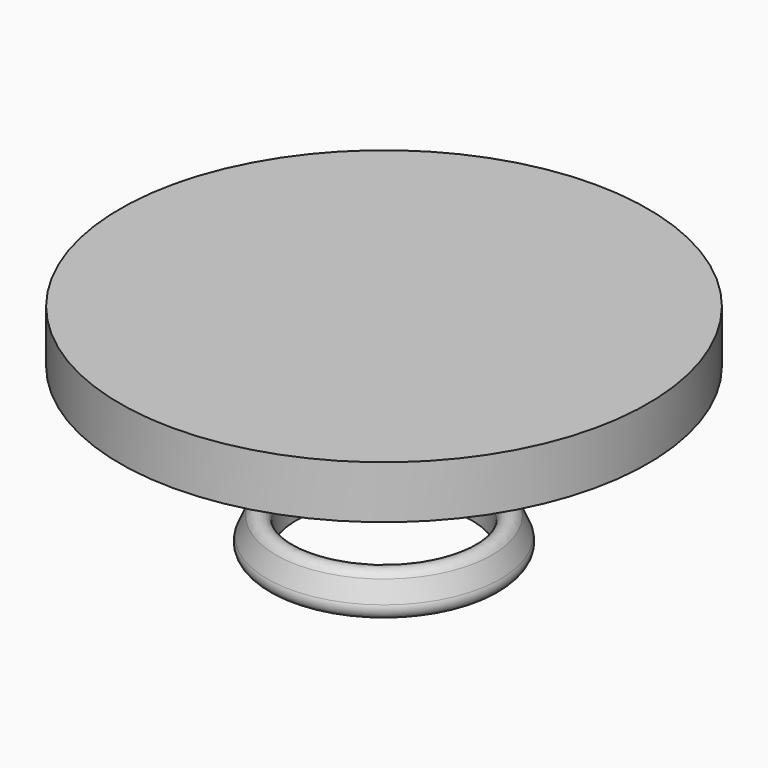
from build123d import *

# Parameters (mm, degrees)
F0_W   = 127
F0_H   = 38.1
F2_R   = 7.62
F2_2_R = 7.62


with BuildPart() as f1:
    # F0 (on Right) → F1 (revolve)
    with BuildSketch(Plane.YZ):
        Polygon((0, 8.3), (0, 0), (35.485, 0), (31.75, 8.3), align=None)
        Polygon((31.75, 8.3), (35.485, 0), (63.5, 0), (63.5, 38.1), (0, 38.1), (0, 8.3), align=None)
        Polygon((63.5, 0), (35.485, 0), (63.5, -62.2555555556), align=None)
        with Locations((127, 19.05)):
            Rectangle(F0_W, F0_H)
    revolve(axis=Axis((0, 0, 4.15), (0, 0, 1)))

    # F2#2
    f2_2_edges = [f1.edges().sort_by_distance(p)[0] for p in [
        (0, -35.485, 0),
        (0, -63.5, -62.255556),
    ]]
    fillet(f2_2_edges, radius=F2_2_R)


with BuildPart() as f1b:
    # F0 (on Right) → F1, piece 2 (revolve)
    with BuildSketch(Plane.YZ):
        Polygon((88.9, -118.7), (63.5, -62.2555555556), (63.5, -118.7), align=None)
    revolve(axis=Axis((0, 0, 4.15), (0, 0, 1)))

    # F2
    f2_edges = [f1b.edges().sort_by_distance(p)[0] for p in [
        (0, -88.9, -118.7),
        (0, -63.5, -62.255556),
    ]]
    fillet(f2_edges, radius=F2_R)


solid = Compound([f1.part, f1b.part])
